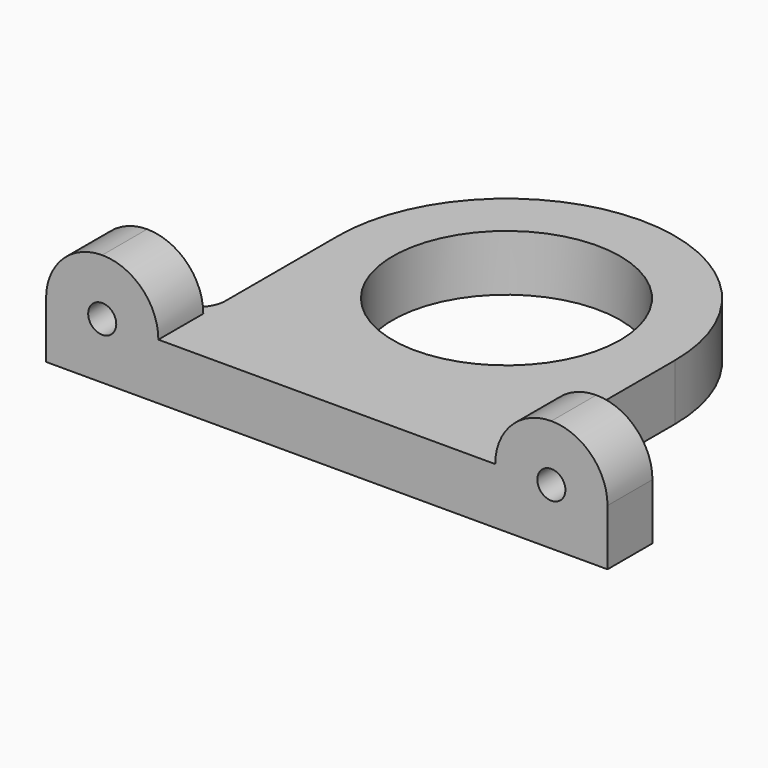
from build123d import *

# Parameters (mm, degrees)
F0_W        = 60
F0_H        = 70
F0_R        = 20.25
F1_DEPTH    = 10
F2_W        = 10
F2_H        = 10
F3_DEPTH    = 20
F4_W        = 10
F4_H        = 10
F5_DEPTH    = 20
F6_R        = 2.5
F7_DEPTH    = 25
F8_T1_DEPTH = 10
F9_R        = 29.99999
F10_R       = 9.99999


# Not quite as in the source:
# - a fillet or chamfer that OpenCascade refuses, or shapes differently, is made with other operations: its cross-section is extruded or revolved along the edge and cut away or added
# - a fillet or chamfer is up to 0.001 mm smaller than in the source, because OpenCascade refuses the exact size


with BuildPart() as f1:
    # F0 (on Top) → F1 (new body)
    with BuildSketch(Plane.XY):
        with Locations((-30.4994795086, -31.9724321365)):
            Rectangle(F0_W, F0_H)
        with Locations((-30.4994795086, -26.9724321365)):
            Circle(F0_R, mode=Mode.SUBTRACT)
    extrude(amount=F1_DEPTH)

    # F2 (on face) → F3 (join)
    with BuildSketch(Plane.YZ.offset(-0.4994795086)):
        with Locations((-61.9724321365, 5)):
            Rectangle(F2_W, F2_H)
        with Locations((-61.9724321365, 15)):
            Rectangle(F2_W, F2_H)
    extrude(amount=F3_DEPTH)

    # F4 (on face) → F5 (join)
    with BuildSketch(Plane(origin=(-60.4994795086, 0, 0), x_dir=(0, -1, 0), z_dir=(-1, 0, 0))):
        with Locations((61.9724321365, 5)):
            Rectangle(F4_W, F4_H)
        with Locations((61.9724321365, 15)):
            Rectangle(F4_W, F4_H)
    extrude(amount=F5_DEPTH)

    # F6 (on face) → F7 (cut)
    with BuildSketch(Plane.XZ.offset(66.9724321365)):
        with Locations((-70.4994795086, 10)):
            Circle(F6_R)
        with Locations((9.5005204914, 10)):
            Circle(F6_R)
    extrude(amount=-F7_DEPTH, mode=Mode.SUBTRACT)

    # F8: fillet of radius 5 on 4 edges, made by hand

    # F8_s2 → F8_t1 (join)
    with BuildSketch(Plane.XY):
        with BuildLine():
            ThreePointArc((-60.4990795086, -51.9714664511), (-61.9639456027, -55.5079660425), (-65.5004451941, -56.9728321365))
            Line((-65.5004451941, -56.9728321365), (-65.5004451941, -57.4729687051))
            ThreePointArc((-65.5004451941, -57.4729687051), (-62.9999623514, -57.4725687051), (-60.4994795086, -57.4725687051))
            Line((-60.4994795086, -57.4725687051), (-59.9993429401, -56.9724321365))
            ThreePointArc((-59.9993429401, -56.9724321365), (-59.9993429401, -54.4719492938), (-59.9989429401, -51.9714664511))
            Line((-59.9989429401, -51.9714664511), (-60.4990795086, -51.9714664511))
        make_face()
        with BuildLine():
            ThreePointArc((-0.4998795086, -51.9714664511), (0.9649865854, -55.5079660425), (4.5014861768, -56.9728321365))
            Line((4.5014861768, -56.9728321365), (4.5014861768, -57.4729687051))
            ThreePointArc((4.5014861768, -57.4729687051), (2.0010033341, -57.4725687051), (-0.4994795086, -57.4725687051))
            Line((-0.4994795086, -57.4725687051), (-0.9996160772, -56.9724321365))
            ThreePointArc((-0.9996160772, -56.9724321365), (-0.9996160772, -54.4719492938), (-1.0000160772, -51.9714664511))
            Line((-1.0000160772, -51.9714664511), (-0.4998795086, -51.9714664511))
        make_face()
    extrude(amount=F8_T1_DEPTH)

    # F9 (radius 30 in the source; OpenCascade refuses exactly that, so slightly less here)
    f9_edges = [f1.edges().sort_by_distance(p)[0] for p in [
        (-60.49948, 3.027568, 5),
        (-0.49948, 3.027568, 5),
    ]]
    fillet(f9_edges, radius=F9_R)

    # F10 (radius 10 in the source; OpenCascade refuses exactly that, so slightly less here)
    f10_edges = [f1.edges().sort_by_distance(p)[0] for p in [
        (19.50052, -61.972432, 20),
        (-80.49948, -61.972432, 20),
        (-60.49948, -61.972432, 20),
        (-0.49948, -61.972432, 20),
    ]]
    fillet(f10_edges, radius=F10_R)


solid = f1.part
